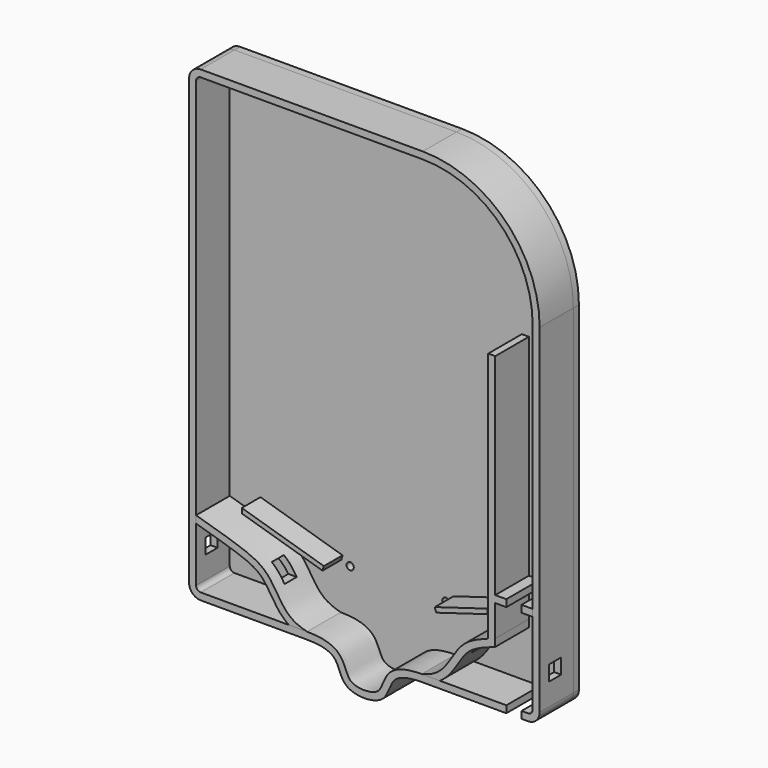
from build123d import *

# Parameters (mm, degrees)
F1_DEPTH  = 3
F3_DEPTH  = 18
F4_DEPTH  = 10
F5_DEPTH  = 18
F7_DEPTH  = 3
F8_W      = 6.5
F8_H      = 6.5
F9_DEPTH  = 150.0010001
F10_DEPTH = 150.0010001
F11_W     = 6.5
F11_H     = 18
F12_DEPTH = 42.9669266491
F13_R     = 1.55
F14_DEPTH = 3.0010001


# Not quite as in the source:
# - ends of sketch curves that miss each other by under 0.0002 mm in the source are joined
# - the dataset's text gives a spline's control points without its knots; the knots are read off the source's solid


with BuildPart() as f1:
    # F0 (on Front) → F1 (new body)
    with BuildSketch(Plane.XZ):
        with BuildLine():
            Line((25, 100), (-70, 100))
            ThreePointArc((-70, 100), (-73.5355339059, 98.5355339059), (-75, 95))
            Line((-75, 95), (-75, -95))
            ThreePointArc((-75, -95), (-73.5355339059, -98.5355339059), (-70, -100))
            Line((-70, -100), (-25, -100))
            add(Edge.make_bspline(
                [(-25, -100), (-20.6615807122, -100), (-10.7939809433, -100.770920602), (-10.3962247958, -114.7727270635), (10.4279303974, -114.7727270635), (10.6655785762, -100.770920602), (20.9708595623, -100), (25, -100)],
                knots=[0, 0, 0, 0, 0.2020990466, 0.3887225818, 0.6112774182, 0.7979009534, 1, 1, 1, 1], degree=3))
            Line((25, -100), (70, -100))
            ThreePointArc((70, -100), (73.5355339059, -98.5355339059), (75, -95))
            Line((75, -95), (75, 50))
            ThreePointArc((75, 50), (60.3553390593, 85.3553390593), (25, 100))
        make_face()
        with BuildLine():
            ThreePointArc((25, 97), (58.2340187158, 83.2340187158), (72, 50))
            Line((72, 50), (72, -95))
            ThreePointArc((72, -95), (71.4142135624, -96.4142135624), (70, -97))
            Line((70, -97), (25, -97))
            add(Edge.make_bspline(
                [(-25, -97), (-24.3005920461, -97), (-22.8475778775, -97.019902158), (-20.5750256034, -97.155072623), (-18.2702104732, -97.4464793332), (-15.985550765, -97.9565503654), (-14.1360130752, -98.6358304265), (-12.7227011231, -99.3961183655), (-11.8798620267, -99.9792382135), (-11.2437249363, -100.5175580629), (-10.7859315829, -100.9631562176), (-10.3692522627, -101.4322261396), (-9.8739446655, -102.068901408), (-9.3530827296, -102.8760888798), (-8.6802194269, -104.1475173706), (-8.0438074166, -105.6538682862), (-7.3912137089, -107.2337391544), (-6.8453212241, -108.2785616486), (-6.3877665701, -108.9261371503), (-6.0894883425, -109.2600602336), (-5.8330193874, -109.4951865243), (-5.6315770879, -109.6555558274), (-5.3964116269, -109.8169593356), (-5.0345944607, -110.0319264035), (-4.4975693595, -110.2907081887), (-3.735904763, -110.5652710439), (-2.8802869246, -110.7898393444), (-1.6459905056, -111.0108211805), (0.012305506, -111.1253632538), (1.6685219906, -111.0108155461), (2.8985385847, -110.7901284112), (3.7495655038, -110.566071103), (4.5051857153, -110.2925228137), (5.0359264642, -110.0352965732), (5.3920458208, -109.8222492594), (5.6226470571, -109.6627081278), (5.8193758193, -109.5046449415), (6.0699699221, -109.2725114463), (6.3617933268, -108.9418385637), (6.8111698988, -108.2968051284), (7.3500217939, -107.2490762941), (8.0004416415, -105.6575559508), (8.6459220446, -104.1360192193), (9.3374549288, -102.8518515479), (9.8754424023, -102.0381971046), (10.3873024899, -101.3986714387), (10.8175721352, -100.9289298047), (11.2892922048, -100.4845047538), (11.9428171147, -99.9498043253), (12.8054026984, -99.3732115055), (14.2463101038, -98.6231758721), (16.1247982656, -97.9524597082), (18.4312543613, -97.4461503108), (20.7322762108, -97.1554882085), (22.9603634866, -97.0200474384), (24.3462218651, -97), (25, -97)],
                knots=[0, 0, 0, 0, 0.03125, 0.0625, 0.09375, 0.125, 0.15625, 0.171875, 0.1875, 0.1953125, 0.203125, 0.2109375, 0.21875, 0.234375, 0.25, 0.28125, 0.3125, 0.34375, 0.359375, 0.375, 0.3828125, 0.390625, 0.3984375, 0.40625, 0.421875, 0.4375, 0.453125, 0.46875, 0.5, 0.53125, 0.546875, 0.5625, 0.578125, 0.59375, 0.6015625, 0.609375, 0.6171875, 0.625, 0.640625, 0.65625, 0.6875, 0.71875, 0.75, 0.765625, 0.78125, 0.7890625, 0.796875, 0.8046875, 0.8125, 0.828125, 0.84375, 0.875, 0.90625, 0.9375, 0.96875, 1, 1, 1, 1], degree=3))
            Line((-25, -97), (-70, -97))
            ThreePointArc((-70, -97), (-71.4142135624, -96.4142135624), (-72, -95))
            Line((-72, -95), (-72, 95))
            ThreePointArc((-72, 95), (-71.4142135624, 96.4142135624), (-70, 97))
            Line((-70, 97), (25, 97))
        make_face(mode=Mode.SUBTRACT)
    extrude(amount=-F1_DEPTH)

    # F8 (on face) → F10 (cut, through all)
    with BuildSketch(Plane.YZ.offset(75)):
        with Locations((-9.75, -82.25)):
            Rectangle(F8_W, F8_H)
    extrude(amount=-F10_DEPTH, mode=Mode.SUBTRACT)


with BuildPart() as f3:
    # F0 (on Front) → F3 (new body)
    with BuildSketch(Plane.XZ):
        with BuildLine():
            Line((25, 100), (-70, 100))
            ThreePointArc((-70, 100), (-73.5355339059, 98.5355339059), (-75, 95))
            Line((-75, 95), (-75, -95))
            ThreePointArc((-75, -95), (-73.5355339059, -98.5355339059), (-70, -100))
            Line((-70, -100), (-25, -100))
            add(Edge.make_bspline(
                [(-25, -100), (-20.6615807122, -100), (-10.7939809433, -100.770920602), (-10.3962247958, -114.7727270635), (10.4279303974, -114.7727270635), (10.6655785762, -100.770920602), (20.9708595623, -100), (25, -100)],
                knots=[0, 0, 0, 0, 0.2020990466, 0.3887225818, 0.6112774182, 0.7979009534, 1, 1, 1, 1], degree=3))
            Line((25, -100), (70, -100))
            ThreePointArc((70, -100), (73.5355339059, -98.5355339059), (75, -95))
            Line((75, -95), (75, 50))
            ThreePointArc((75, 50), (60.3553390593, 85.3553390593), (25, 100))
        make_face()
        with BuildLine():
            ThreePointArc((25, 97), (58.2340187158, 83.2340187158), (72, 50))
            Line((72, 50), (72, -95))
            ThreePointArc((72, -95), (71.4142135624, -96.4142135624), (70, -97))
            Line((70, -97), (25, -97))
            add(Edge.make_bspline(
                [(-25, -97), (-24.3005920461, -97), (-22.8475778775, -97.019902158), (-20.5750256034, -97.155072623), (-18.2702104732, -97.4464793332), (-15.985550765, -97.9565503654), (-14.1360130752, -98.6358304265), (-12.7227011231, -99.3961183655), (-11.8798620267, -99.9792382135), (-11.2437249363, -100.5175580629), (-10.7859315829, -100.9631562176), (-10.3692522627, -101.4322261396), (-9.8739446655, -102.068901408), (-9.3530827296, -102.8760888798), (-8.6802194269, -104.1475173706), (-8.0438074166, -105.6538682862), (-7.3912137089, -107.2337391544), (-6.8453212241, -108.2785616486), (-6.3877665701, -108.9261371503), (-6.0894883425, -109.2600602336), (-5.8330193874, -109.4951865243), (-5.6315770879, -109.6555558274), (-5.3964116269, -109.8169593356), (-5.0345944607, -110.0319264035), (-4.4975693595, -110.2907081887), (-3.735904763, -110.5652710439), (-2.8802869246, -110.7898393444), (-1.6459905056, -111.0108211805), (0.012305506, -111.1253632538), (1.6685219906, -111.0108155461), (2.8985385847, -110.7901284112), (3.7495655038, -110.566071103), (4.5051857153, -110.2925228137), (5.0359264642, -110.0352965732), (5.3920458208, -109.8222492594), (5.6226470571, -109.6627081278), (5.8193758193, -109.5046449415), (6.0699699221, -109.2725114463), (6.3617933268, -108.9418385637), (6.8111698988, -108.2968051284), (7.3500217939, -107.2490762941), (8.0004416415, -105.6575559508), (8.6459220446, -104.1360192193), (9.3374549288, -102.8518515479), (9.8754424023, -102.0381971046), (10.3873024899, -101.3986714387), (10.8175721352, -100.9289298047), (11.2892922048, -100.4845047538), (11.9428171147, -99.9498043253), (12.8054026984, -99.3732115055), (14.2463101038, -98.6231758721), (16.1247982656, -97.9524597082), (18.4312543613, -97.4461503108), (20.7322762108, -97.1554882085), (22.9603634866, -97.0200474384), (24.3462218651, -97), (25, -97)],
                knots=[0, 0, 0, 0, 0.03125, 0.0625, 0.09375, 0.125, 0.15625, 0.171875, 0.1875, 0.1953125, 0.203125, 0.2109375, 0.21875, 0.234375, 0.25, 0.28125, 0.3125, 0.34375, 0.359375, 0.375, 0.3828125, 0.390625, 0.3984375, 0.40625, 0.421875, 0.4375, 0.453125, 0.46875, 0.5, 0.53125, 0.546875, 0.5625, 0.578125, 0.59375, 0.6015625, 0.609375, 0.6171875, 0.625, 0.640625, 0.65625, 0.6875, 0.71875, 0.75, 0.765625, 0.78125, 0.7890625, 0.796875, 0.8046875, 0.8125, 0.828125, 0.84375, 0.875, 0.90625, 0.9375, 0.96875, 1, 1, 1, 1], degree=3))
            Line((-25, -97), (-70, -97))
            ThreePointArc((-70, -97), (-71.4142135624, -96.4142135624), (-72, -95))
            Line((-72, -95), (-72, 95))
            ThreePointArc((-72, 95), (-71.4142135624, 96.4142135624), (-70, 97))
            Line((-70, 97), (25, 97))
        make_face(mode=Mode.SUBTRACT)
    extrude(amount=F3_DEPTH)


with BuildPart() as f4:
    # F2 (on Front) → F4 (new body)
    with BuildSketch(Plane.XZ):
        Polygon((46.3427752463, -68.5295255307), (23.7287843341, -75.2875918635), (24.3014483328, -77.2038527916), (46.3427752463, -70.6169239332), align=None)
    extrude(amount=F4_DEPTH)


with BuildPart() as f4b:
    # F2 (on Front) → F4, piece 2 (new body)
    with BuildSketch(Plane.XZ):
        Polygon((-24.3014483328, -77.2038527916), (-23.7287843341, -75.2875918635), (-58.8374363, -64.7955650576), (-58.8374363, -66.8829634601), align=None)
    extrude(amount=F4_DEPTH)


with BuildPart() as f5:
    # F2 (on Front) → F5 (new body)
    with BuildSketch(Plane.XZ):
        with BuildLine():
            add(Edge.make_bspline(
                [(-72, -68.5958850782), (-68.746955986, -69.5440934623), (-61.6178328083, -71.6220960385), (-46.3943462387, -76.2968100482), (-39.8285361724, -82.049997427), (-34.8388000594, -91.3712637708), (-29.6068278015, -95.5392485184), (-26.1356954498, -96.5332723648), (-24.5021813041, -97)],
                knots=[0, 0, 0, 0, 0.1816291377, 0.3980781468, 0.5604572014, 0.7358779539, 0.8758516034, 1, 1, 1, 1], degree=3))
            Line((-72, -68.5958850782), (-71.9999999998, -71.7207533204))
            add(Edge.make_bspline(
                [(-71.9999999998, -71.7207533204), (-71.1593506619, -71.9658578038), (-69.1892465946, -72.5407390924), (-66.5364227542, -73.3203665785), (-63.9945448322, -74.0756258986), (-61.9662256671, -74.682593981), (-59.8196928713, -75.3318616745), (-56.884749776, -76.24828087), (-53.943663458, -77.2367146748), (-51.2286365845, -78.2777215699), (-49.6784736007, -78.9427504134), (-48.5594330954, -79.4763263745), (-47.5363759272, -80.0056119863), (-46.42054435, -80.6676749916), (-45.2826627901, -81.4857807614), (-44.2796240259, -82.3620321648), (-43.3449939882, -83.3457396598), (-42.4304306777, -84.4817146192), (-41.4792435181, -85.8340473089), (-40.4957570405, -87.343080275), (-39.4829175587, -88.9377793508), (-38.4306733498, -90.5580820099), (-37.5071791271, -91.8817345745), (-36.7218758472, -92.9030123371), (-35.9049406213, -93.8805278553), (-34.8516608448, -94.9853189374), (-33.5751583037, -96.0992422127), (-32.7089222668, -96.7260338888), (-32.2939694222, -96.9999968107)],
                knots=[0.0156196017, 0.0156196017, 0.0156196017, 0.0156196017, 0.0625, 0.125, 0.15625, 0.1875, 0.21875, 0.25, 0.3125, 0.34375, 0.375, 0.390625, 0.40625, 0.4375, 0.46875, 0.5, 0.53125, 0.5625, 0.59375, 0.625, 0.65625, 0.6875, 0.71875, 0.734375, 0.75, 0.78125, 0.8125, 0.8404968354, 0.8404968354, 0.8404968354, 0.8404968354], degree=3))
            Line((-32.2939694222, -96.9999968107), (-24.5021813041, -97))
        make_face()
    extrude(amount=F5_DEPTH)


with BuildPart() as f5b:
    # F2 (on Front) → F5, piece 2 (new body)
    with BuildSketch(Plane.XZ):
        with BuildLine():
            add(Edge.make_bspline(
                [(56.0000191512, -76.5536411472), (55.0775206084, -76.8614515092), (53.444172632, -77.4282315246), (51.2286365845, -78.2777215699), (49.6784736007, -78.9427504134), (48.5594330954, -79.4763263745), (47.5363759272, -80.0056119863), (46.42054435, -80.6676749916), (45.2826627901, -81.4857807614), (44.2796240259, -82.3620321648), (43.3449939882, -83.3457396598), (42.4304306777, -84.4817146192), (41.4792435181, -85.8340473089), (40.4957570405, -87.343080275), (39.4829175587, -88.9377793508), (38.4306733498, -90.5580820099), (37.5071791271, -91.8817345745), (36.7218758472, -92.9030123371), (35.9049406213, -93.8805278553), (34.8516608448, -94.9853189374), (33.5592141306, -96.1131556872), (32.6758578563, -96.749913316), (32.2436817697, -97.0330713347)],
                knots=[0.2729965876, 0.2729965876, 0.2729965876, 0.2729965876, 0.3125, 0.34375, 0.375, 0.390625, 0.40625, 0.4375, 0.46875, 0.5, 0.53125, 0.5625, 0.59375, 0.625, 0.65625, 0.6875, 0.71875, 0.734375, 0.75, 0.78125, 0.8125, 0.8416271874, 0.8416271874, 0.8416271874, 0.8416271874], degree=3))
            Line((56.0000191512, -76.5536411472), (56, -73.3950051509))
            add(Edge.make_bspline(
                [(56, -73.3950051509), (54.9931782113, -73.7226683624), (53.9859090273, -74.0626004291), (53, -74.41396003)],
                knots=[0.2597850123, 0.2597850123, 0.2597850123, 0.2597850123, 0.3017925269, 0.3017925269, 0.3017925269, 0.3017925269], degree=3))
            add(Edge.make_bspline(
                [(53, -74.41396003), (50.7401933224, -75.2193130093), (44.9708520117, -77.5441243838), (39.8285361724, -82.049997427), (34.8388000594, -91.3712637708), (29.6068278015, -95.5392485184), (26.1356954498, -96.5332723648), (24.5021813041, -97)],
                knots=[0.3017925269, 0.3017925269, 0.3017925269, 0.3017925269, 0.3980781468, 0.5604572014, 0.7358779539, 0.8758516034, 1, 1, 1, 1], degree=3))
            Line((24.5021813041, -97), (32.2436817697, -97.0330713347))
        make_face()
        with BuildLine():
            add(Edge.make_bspline(
                [(56, -73.3950051509), (54.9931782113, -73.7226683624), (53.9859090273, -74.0626004291), (53, -74.41396003)],
                knots=[0.2597850123, 0.2597850123, 0.2597850123, 0.2597850123, 0.3017925269, 0.3017925269, 0.3017925269, 0.3017925269], degree=3))
            Line((56, -73.3950051509), (56, -60.0330733509))
            Line((56, -60.0330733509), (72, -60.0330733509))
            Line((72, -60.0330733509), (72, -57.0330733509))
            Line((72, -57.0330733509), (56, -57.0330733509))
            Line((56, -57.0330733509), (56, 32.9669266491))
            Line((56, 32.9669266491), (53, 32.9669266491))
            Line((53, 32.9669266491), (53, -74.41396003))
        make_face()
    extrude(amount=F5_DEPTH)


with BuildPart() as f7:
    # F6 (on Front) → F7 (new body)
    with BuildSketch(Plane.XZ):
        with BuildLine():
            Line((25, 100), (-70, 100))
            ThreePointArc((-70, 100), (-73.5355339059, 98.5355339059), (-75, 95))
            Line((-75, 95), (-75, -95))
            ThreePointArc((-75, -95), (-73.5355339059, -98.5355339059), (-70, -100))
            Line((-70, -100), (-25, -100))
            add(Edge.make_bspline(
                [(-25, -100), (-20.6615807122, -100), (-10.7939809433, -100.770920602), (-10.3962247958, -114.7727270635), (10.4279303974, -114.7727270635), (10.6655785762, -100.770920602), (20.9708595623, -100), (25, -100)],
                knots=[0, 0, 0, 0, 0.2020990466, 0.3887225818, 0.6112774182, 0.7979009534, 1, 1, 1, 1], degree=3))
            Line((25, -100), (70, -100))
            ThreePointArc((70, -100), (73.5355339059, -98.5355339059), (75, -95))
            Line((75, -95), (75, 50))
            ThreePointArc((75, 50), (60.3553390593, 85.3553390593), (25, 100))
        make_face()
    extrude(amount=-F7_DEPTH)

    # F13 (on face) → F14 (cut, through all)
    with BuildSketch(Plane.XZ):
        with Locations((-20.4689264766, -78.349180789)):
            Circle(F13_R)
        with Locations((20.4689264766, -78.349180789)):
            Circle(F13_R)
    extrude(amount=-F14_DEPTH, mode=Mode.SUBTRACT)


with BuildPart() as f9_tool:
    # F8 (on face) → F9 (new body, through all)
    with BuildSketch(Plane.YZ.offset(75)):
        with Locations((-9.75, -82.25)):
            Rectangle(F8_W, F8_H)
    extrude(amount=-F9_DEPTH)


with BuildPart() as f3_1:
    add(f3.part)

    # F9: cut by f9_tool
    add(f9_tool.part, mode=Mode.SUBTRACT)


with BuildPart() as f5_1:
    add(f5.part)

    # F9: cut by f9_tool
    add(f9_tool.part, mode=Mode.SUBTRACT)


with BuildPart() as f5b_1:
    add(f5b.part)

    # F9: cut by f9_tool
    add(f9_tool.part, mode=Mode.SUBTRACT)


with BuildPart() as f12_tool:
    # F11 (on face) → F12 (new body, through all)
    with BuildSketch(Plane(origin=(0, 0, -100), x_dir=(1, 0, 0), z_dir=(0, 0, -1))):
        with Locations((64, 9)):
            Rectangle(F11_W, F11_H)
    extrude(amount=-F12_DEPTH)


with BuildPart() as f3_2:
    add(f3_1.part)

    # F12: cut by f12_tool
    add(f12_tool.part, mode=Mode.SUBTRACT)


with BuildPart() as f5b_2:
    add(f5b_1.part)

    # F12: cut by f12_tool
    add(f12_tool.part, mode=Mode.SUBTRACT)


solid = Compound([f1.part, f4.part, f4b.part, f7.part, f5_1.part, f3_2.part, f5b_2.part])
